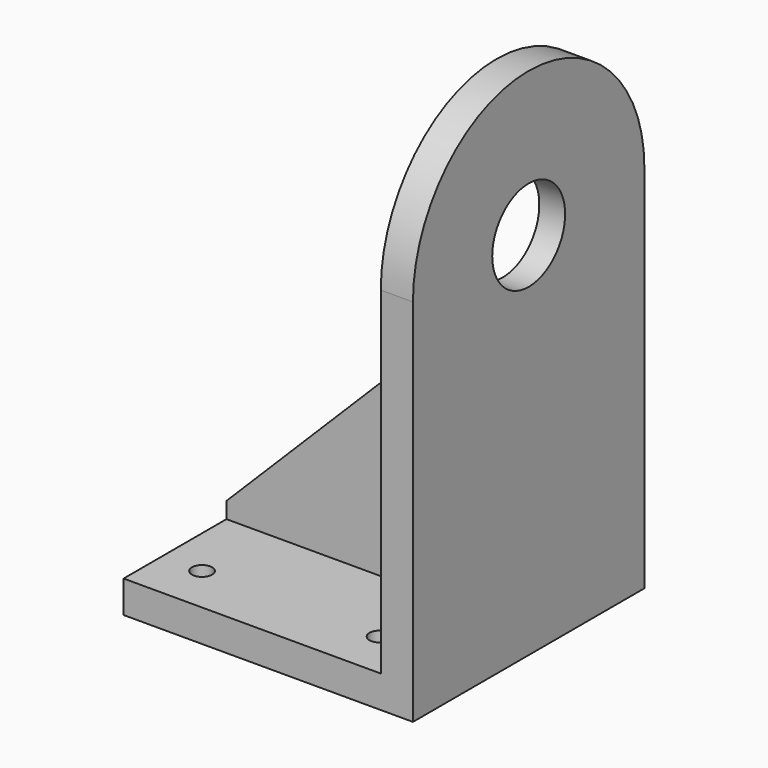
from build123d import *

# Parameters (mm, degrees)
F1_DEPTH       = 12.7
F2_D           = 36
F2_DEPTH       = 36
F2_CBORE_D     = 65
F2_CBORE_DEPTH = 2.5
F2_TIP         = 10.8154911425
F4_D           = 4.4
F4_DEPTH       = 10
F4_TIP         = 1.3218933619
F5_W           = 114.3
F5_H           = 12.7
F6_DEPTH       = 101.6
F7_W           = 101.6
F7_H           = 76.2
F8_DEPTH       = 6.35
F9_SIZE        = 69.85
F11_D          = 7.9375


# Not quite as in the source:
# - a length typed as a fraction of an inch, garbled in the dataset ("3 / 203.2 mm" for 3/8 in), is restored


with BuildPart() as f1:
    # F0 (on Right) → F1 (new body)
    with BuildSketch(Plane.YZ):
        with BuildLine():
            Line((57.15, -146.05), (57.15, 0))
            ThreePointArc((57.15, 0), (0, 57.15), (-57.15, 0))
            Line((-57.15, 0), (-57.15, -146.05))
            Line((-57.15, -146.05), (57.15, -146.05))
        make_face()
    extrude(amount=F1_DEPTH)

    # F2
    with Locations(Plane(origin=(0, 0, 0), x_dir=(0, 1, 0), z_dir=(-1, 0, 0))):
        with Locations((0, 0)):
            CounterBoreHole(F2_D / 2, F2_CBORE_D / 2, F2_CBORE_DEPTH, depth=F2_DEPTH)
            with Locations((0, 0, -(F2_DEPTH + F2_TIP / 2))):  # 118° drill point
                Cone(0, F2_D / 2, F2_TIP, mode=Mode.SUBTRACT)

    # F4
    with Locations(Plane(origin=(0, 0, 0), x_dir=(0, 1, 0), z_dir=(-1, 0, 0))):
        with Locations((35.814, -13.03522997), (35.814, 13.03522997), (-35.814, -13.03522997), (-35.814, 13.03522997)):
            Hole(F4_D / 2, depth=F4_DEPTH)
            with Locations((0, 0, -(F4_DEPTH + F4_TIP / 2))):  # 118° drill point
                Cone(0, F4_D / 2, F4_TIP, mode=Mode.SUBTRACT)

    # F5 (on face) → F6 (join)
    with BuildSketch(Plane.YZ):
        with Locations((0, -139.7)):
            Rectangle(F5_W, F5_H)
    extrude(amount=-F6_DEPTH)

    # F7 (on Front) → F8 (join, symmetric)
    with BuildSketch(Plane.XZ):
        with Locations((-50.8, -95.25)):
            Rectangle(F7_W, F7_H)
    extrude(amount=F8_DEPTH, both=True)

    # F9
    f9_edges = [f1.edges().sort_by_distance(p)[0] for p in [
        (-101.6, 0, -57.15),
    ]]
    chamfer(f9_edges, length=F9_SIZE)

    # F11 (through all)
    with Locations(Plane(origin=(0, 0, -146.05), x_dir=(1, 0, 0), z_dir=(0, 0, -1))):
        with Locations((-85.852, 38.1), (-15.748, 38.1), (-85.852, -38.1), (-15.748, -38.1)):
            Hole(F11_D / 2)


solid = f1.part
